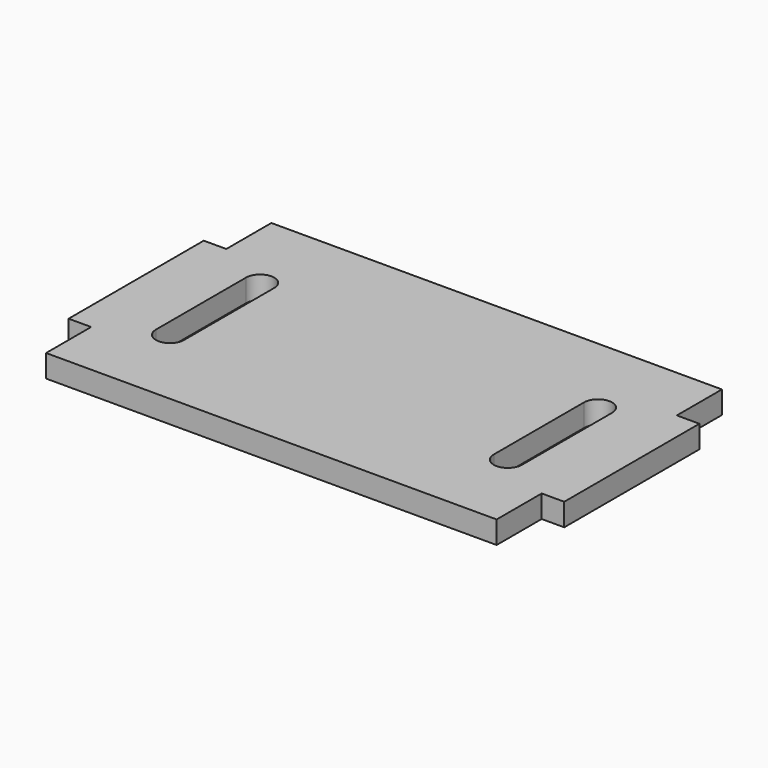
from build123d import *

# Parameters (mm, degrees)
F0_W     = 40
F0_H     = 25
F1_DEPTH = 2
F2_W     = 2
F2_H     = 15
F3_DEPTH = 2
F5_DEPTH = 2.001


# Not quite as in the source:
# - a pattern or mirror of a feature is missing from the dataset's text; its kind, count and spacing are read off the source's solid


with BuildPart() as f1:
    # F0 (on Top) → F1 (new body)
    with BuildSketch(Plane.XY):
        Rectangle(F0_W, F0_H)
    extrude(amount=F1_DEPTH)

    # F2 (on Top) → F3 (join)
    with BuildSketch(Plane.XY):
        with Locations((-21, 0)):
            Rectangle(F2_W, F2_H)
    f3 = extrude(amount=F3_DEPTH)

    # F3_copies: F3 across plane
    add(f3.mirror(Plane(origin=(0, 0, 0), x_dir=(0, 0, 1), z_dir=(1, 0, 0))))

    # F4 (on face) → F5 (cut, through all)
    with BuildSketch(Plane.XY.offset(2)):
        with BuildLine():
            ThreePointArc((-13.75, 5), (-15, 6.25), (-16.25, 5))
            Line((-16.25, 5), (-16.25, -5))
            ThreePointArc((-16.25, -5), (-15, -6.25), (-13.75, -5))
            Line((-13.75, -5), (-13.75, 5))
        make_face()
    f5 = extrude(amount=-F5_DEPTH, mode=Mode.SUBTRACT)

    # F5_copies: F5 across plane
    add(f5.mirror(Plane(origin=(0, 0, 0), x_dir=(0, 0, 1), z_dir=(1, 0, 0))), mode=Mode.SUBTRACT)


solid = f1.part
